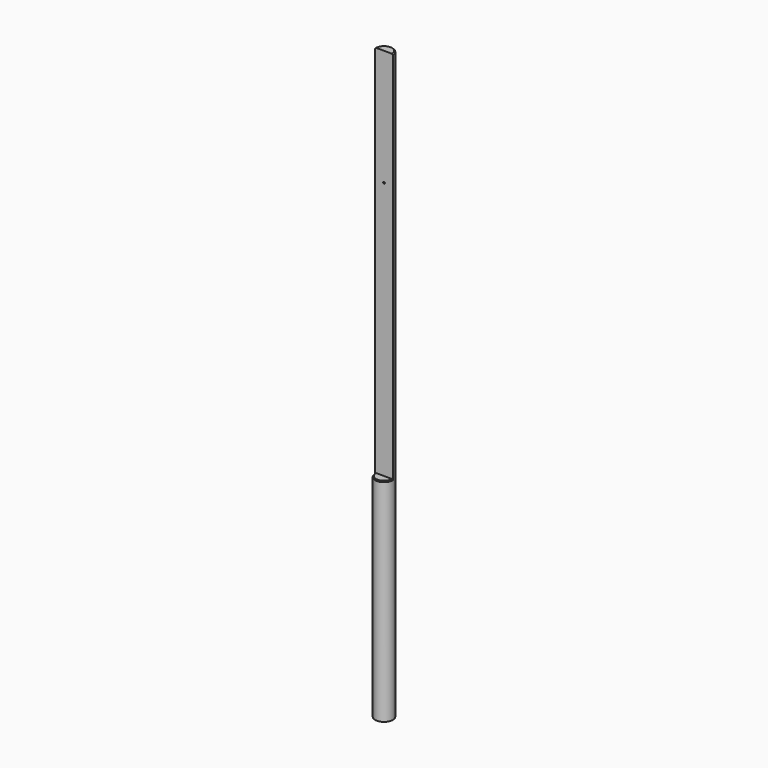
from build123d import *

# Parameters (mm, degrees)
F1_DEPTH    = 1060
F2_DEPTH    = 600
F3_T2_ANGLE = 180
F4_SIZE     = 2.54
F6_D        = 5


# Not quite as in the source:
# - a fillet or chamfer that OpenCascade refuses, or shapes differently, is made with other operations: its cross-section is extruded or revolved along the edge and cut away or added


with BuildPart() as f1:
    # F0 (on Top) → F1 (new body)
    with BuildSketch(Plane.XY):
        with BuildLine():
            Line((-25, 0), (25, 0))
            ThreePointArc((25, 0), (0, 25), (-25, 0))
        make_face()
    extrude(amount=F1_DEPTH)

    # F0 (on Top) → F2 (join)
    with BuildSketch(Plane.XY):
        with BuildLine():
            ThreePointArc((-25, 0), (0, -25), (25, 0))
            Line((25, 0), (-25, 0))
        make_face()
        with BuildLine():
            Line((-25, 0), (25, 0))
            ThreePointArc((25, 0), (0, 25), (-25, 0))
        make_face()
    extrude(amount=-F2_DEPTH)

    # F3: chamfer of 2.54 on 1 edges, made by hand

    # F3_s1 → F3_t2 (revolve, cut)
    with BuildSketch(Plane.XZ):
        Polygon((-25, -2.54), (-22.46, 0), (-25, 0), align=None)
    revolve(axis=Axis((0, 0, 0), (0, 0, 1)), revolution_arc=F3_T2_ANGLE, mode=Mode.SUBTRACT)

    # F4
    f4_edges = [f1.edges().sort_by_distance(p)[0] for p in [
        (0, 25, 1060),
    ]]
    chamfer(f4_edges, length=F4_SIZE)

    # F6 (through all)
    with Locations(Plane.XZ):
        with Locations((0, 730.6740903854)):
            Hole(F6_D / 2)


solid = f1.part
